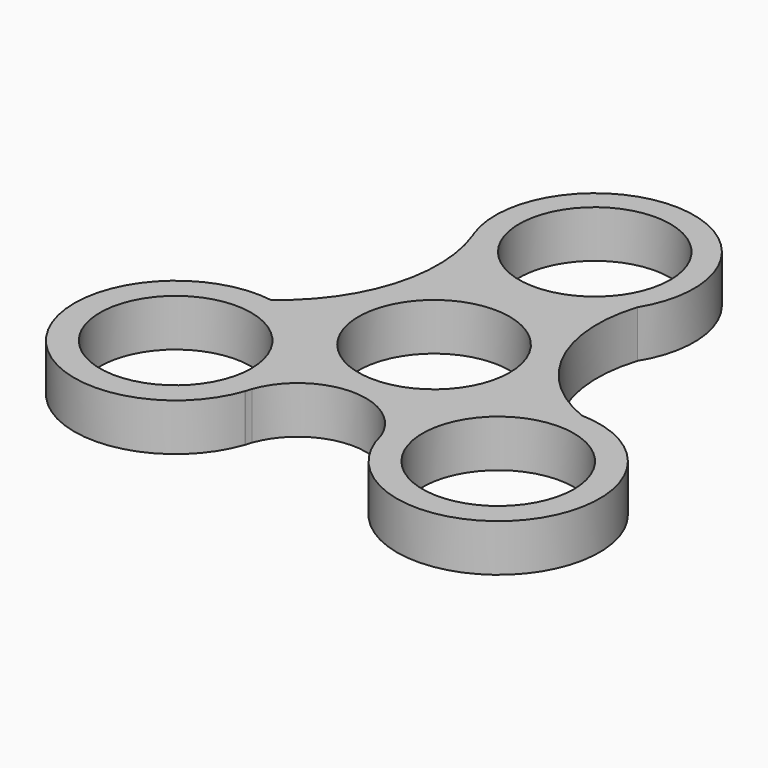
from build123d import *

# Parameters (mm, degrees)
F0_R        = 11.2
F1_DEPTH    = 7
F2_T1_DEPTH = 7.3091738438


# Not quite as in the source:
# - a fillet or chamfer that OpenCascade refuses, or shapes differently, is made with other operations: its cross-section is extruded or revolved along the edge and cut away or added


with BuildPart() as f1:
    # F0 (on Top) → F1 (new body)
    with BuildSketch(Plane.XY):
        with BuildLine():
            ThreePointArc((24.4140649416, -3.1809629834), (13.4871120811, 7.0747385166), (12.5205974964, 22.0294555527))
            ThreePointArc((12.5205974964, 22.0294555527), (1.5158634118, 44.3693332806), (-13.8361222225, 24.7608951415))
            ThreePointArc((-13.8361222225, 24.7608951415), (-13.7078172482, 24.4365570296), (-13.5843298249, 24.1103542803))
            ThreePointArc((-13.5843298249, 24.1103542803), (-13.113174784, 9.1691492017), (-21.7305353918, -3.0457061978))
            ThreePointArc((-21.7305353918, -3.0457061978), (-36.801707194, -25.6538021325), (-9.7868965809, -22.7441236587))
            ThreePointArc((-9.7868965809, -22.7441236587), (-9.6574780237, -22.2857276707), (-9.506618108, -21.8339342105))
            ThreePointArc((-9.506618108, -21.8339342105), (-0.1149775919, -15.1499512762), (9.4355546579, -21.6048620576))
            ThreePointArc((9.4355546579, -21.6048620576), (35.6773528954, -27.6386082592), (24.4140649416, -3.1809629834))
        make_face()
        with Locations((-23.9752419293, -17.876798287)):
            Circle(F0_R, mode=Mode.SUBTRACT)
        Circle(F0_R, mode=Mode.SUBTRACT)
        with Locations((24.0384545177, -18.176259473)):
            Circle(F0_R, mode=Mode.SUBTRACT)
        with Locations((0, 29.7421794385)):
            Circle(F0_R, mode=Mode.SUBTRACT)
    extrude(amount=F1_DEPTH)

    # F2: fillet of radius 1.5 on 1 edges, made by hand

    # F2_s2 → F2_t1 (cut)
    with BuildSketch(Plane.XY.offset(-0.1545869219)):
        with BuildLine():
            ThreePointArc((-9.7727399665, -22.6912544357), (-9.7886409139, -22.7473067601), (-9.8067032425, -22.8027004014))
            Line((-9.8067032425, -22.8027004014), (-9.6647949432, -22.8520369213))
            ThreePointArc((-9.6647949432, -22.8520369213), (-9.6549491563, -22.8224010768), (-9.6447861139, -22.7928747896))
            Line((-9.6447861139, -22.7928747896), (-9.6413873814, -22.7815286112))
            ThreePointArc((-9.6413873814, -22.7815286112), (-9.6346402283, -22.7554279828), (-9.6274353396, -22.7294463591))
            Line((-9.6274353396, -22.7294463591), (-9.7727399665, -22.6912544357))
        make_face()
    extrude(amount=F2_T1_DEPTH, mode=Mode.SUBTRACT)


solid = f1.part
